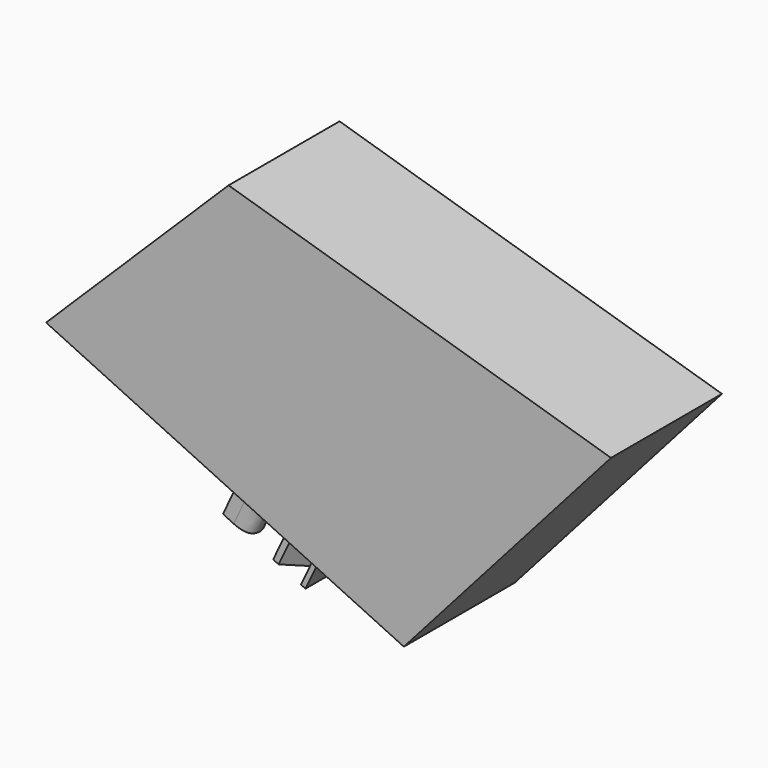
from build123d import *

# Parameters (mm, degrees)
F1_DEPTH     = 50
F2_T         = -2.5
F3_TEXT_SIZE = 23.0710332592
F4_DEPTH     = 25


# Not quite as in the source:
# - Text() gives the source's letters only with a copy of the font that has no kerning and outlines rounded to 1/6400 em; it was checked with that copy


with BuildPart() as f1:
    # F0 (on Front) → F1 (new body)
    with BuildSketch(Plane.XZ):
        Polygon((-208.1390172243, -3.9366418496), (-273.9495933056, -68.8974708319), (-144.9399590492, -129.849165678), (-70.2501833439, -45.611333102), align=None)
    extrude(amount=F1_DEPTH)

    # F2
    f2_openings = [f1.faces().sort_by_distance(p)[0] for p in [
        (-172.134956, 0, -63.345733),
    ]]
    offset(amount=F2_T, openings=f2_openings)

    # F3 (on face) → F4 (join)
    with BuildSketch(Plane(origin=(-76.6024360647, 0, -162.1358074587), x_dir=(0.9041661507, 0, -0.4271809592), z_dir=(-0.4271809592, 0, -0.9041661507))):
        with Locations((-153.2122939825, 16.5350455791)):
            Text('P.N.', F3_TEXT_SIZE, font='Open Sans', text_align=(TextAlign.LEFT, TextAlign.BOTTOM))
    extrude(amount=F4_DEPTH)


solid = f1.part
